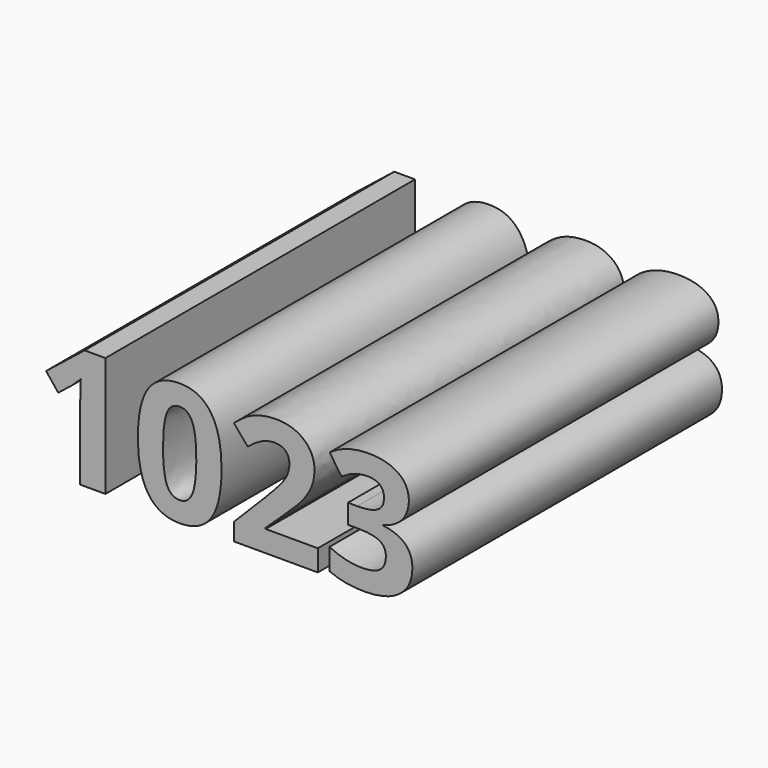
from build123d import *

# Parameters (mm, degrees)
F0_TEXT_SIZE = 10.99864682
F1_DEPTH     = 25.4


# Not quite as in the source:
# - Text() gives the source's letters only with a copy of the font that has no kerning and outlines rounded to 1/6400 em; it was checked with that copy


with BuildPart() as f1:
    # F0 (on Front) → F1 (new body)
    with BuildSketch(Plane.XZ):
        with Locations((-14.7453296318, -5.5407464731)):
            Text('1023', F0_TEXT_SIZE, font='Open Sans', font_style=FontStyle.BOLD, text_align=(TextAlign.LEFT, TextAlign.BOTTOM))
    extrude(amount=F1_DEPTH)


solid = f1.part
